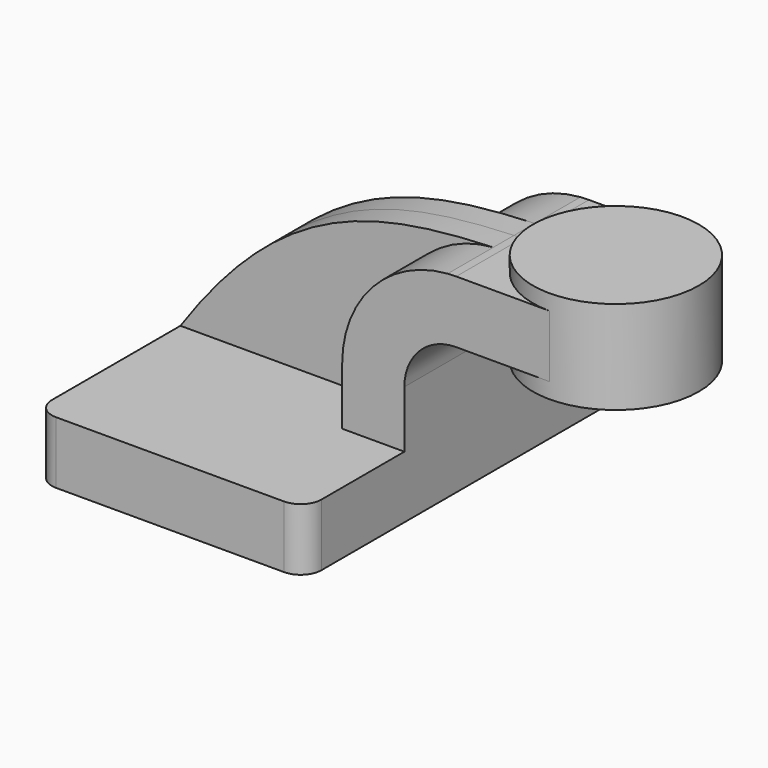
from build123d import *

# Parameters (mm, degrees)
F1_DEPTH = 63.5
F0_W     = 25.4
F0_H     = 19.05
F2_DEPTH = 25.4
F3_DEPTH = 7.9375
F5_R     = 6.35
F6_R     = 6.35
F7_R     = 6.35
F8_R     = 6.35


# Not quite as in the source:
# - a feature names something its author has since deleted; it is built from what else it names


with BuildPart() as f1:
    # F0 (on Front) → F1 (new body, symmetric)
    with BuildSketch(Plane.XZ):
        Polygon((22.225, 9.525), (-41.275, 9.525), (-41.275, -9.525), (41.275, -9.525), (41.275, 9.525), align=None)
    extrude(amount=F1_DEPTH, both=True)

    # F0 (on Front) → F2 (join, symmetric)
    with BuildSketch(Plane.XZ):
        with BuildLine():
            Line((22.225, 27.0002), (22.225, 9.525))
            Line((22.225, 9.525), (41.275, 9.525))
            Line((41.275, 9.525), (41.275, 27.0002))
            ThreePointArc((41.275, 27.0002), (45.9246798487, 38.2255201513), (57.15, 42.8752))
            Line((57.15, 42.8752), (60.325, 42.8752))
            Line((60.325, 42.8752), (60.325, 61.9252))
            Line((60.325, 61.9252), (57.15, 61.9252))
            add(Edge.make_bspline(
                [(54.5418748685, 61.8276792125), (55.4058435477, 61.8626883172), (56.2751659775, 61.8950651933), (57.15, 61.9252)],
                knots=[109.0113637744, 109.0113637744, 109.0113637744, 109.0113637744, 111.5045361635, 111.5045361635, 111.5045361635, 111.5045361635], degree=3))
            ThreePointArc((54.5418748685, 61.8276792125), (31.5487852318, 50.7559030498), (22.225, 27.0002))
        make_face()
        with Locations((73.025, 52.4002)):
            Rectangle(F0_W, F0_H)
    extrude(amount=F2_DEPTH, both=True)

    # F0 (on Front) → F3 (join, symmetric)
    with BuildSketch(Plane.XZ):
        with BuildLine():
            add(Edge.make_bspline(
                [(-41.275, 9.525), (-10.7751676539, 53.7339523615), (16.7657449889, 60.2969426058), (54.5418748685, 61.8276792125)],
                knots=[0, 0, 0, 0, 109.0113637744, 109.0113637744, 109.0113637744, 109.0113637744], degree=3))
            Line((-41.275, 9.525), (22.225, 9.525))
            Line((22.225, 9.525), (22.225, 27.0002))
            ThreePointArc((22.225, 27.0002), (31.5487852318, 50.7559030498), (54.5418748685, 61.8276792125))
        make_face()
    extrude(amount=F3_DEPTH, both=True)

    # F0 (on Front) → F4 (revolve)
    with BuildSketch(Plane.XZ):
        Polygon((85.725, 66.675), (85.725, 61.9252), (85.725, 42.8752), (85.725, 38.1), (111.125, 38.1), (111.125, 66.675), align=None)
    revolve(axis=Axis((85.725, 0, 52.3875), (0, 0, -1)))

    # F5
    f5_edges = [f1.edges().sort_by_distance(p)[0] for p in [
        (41.275, -63.5, 0),
    ]]
    fillet(f5_edges, radius=F5_R)

    # F6
    f6_edges = [f1.edges().sort_by_distance(p)[0] for p in [
        (-41.275, -63.5, 0),
    ]]
    fillet(f6_edges, radius=F6_R)

    # F7
    f7_edges = [f1.edges().sort_by_distance(p)[0] for p in [
        (-41.275, 63.5, 0),
    ]]
    fillet(f7_edges, radius=F7_R)

    # F8
    f8_edges = [f1.edges().sort_by_distance(p)[0] for p in [
        (41.275, 63.5, 0),
    ]]
    fillet(f8_edges, radius=F8_R)


solid = f1.part
